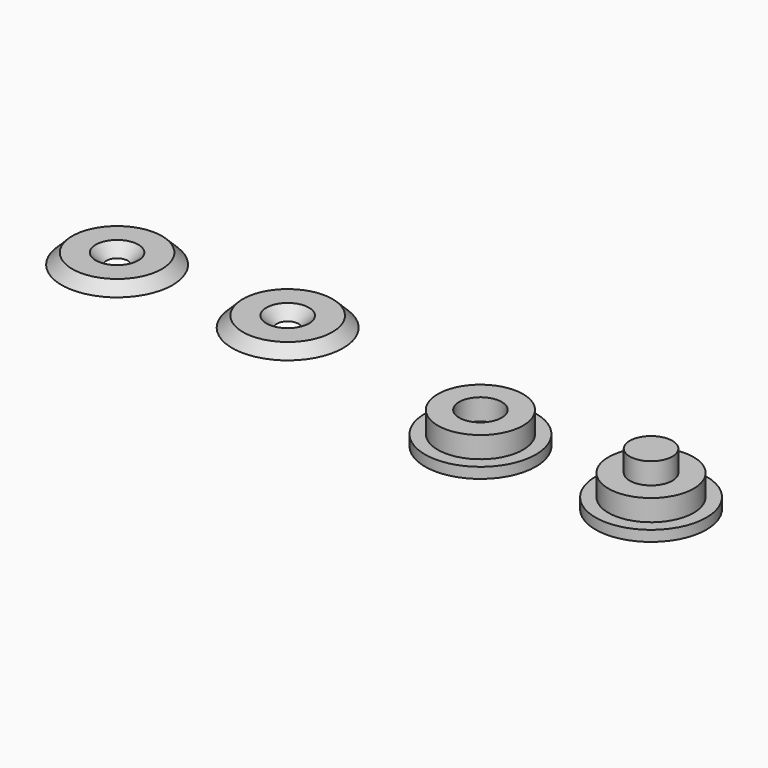
from build123d import *

# Parameters (mm, degrees)
F0_R      = 6.35
F0_R_2    = 3.175
F1_DEPTH  = 3.175
F2_R      = 8.255
F3_DEPTH  = 3.175
F5_R      = 3.175
F6_DEPTH  = 6.35
F8_DEPTH  = 3.175
F10_DEPTH = 6.35
F11_DEPTH = 1.5875
F12_R     = 8.255
F13_DEPTH = 1.5875
F13_TAPER = 45
F14_R     = 3.175
F16_DEPTH = 1.5875


# Not quite as in the source:
# - an extrude whose draft closes it to a point is written as a loft to that point


with BuildPart() as f1:
    # F0 (on Top) → F1 (new body)
    with BuildSketch(Plane.XY):
        Circle(F0_R)
        Circle(F0_R_2, mode=Mode.SUBTRACT)
    extrude(amount=F1_DEPTH)

    # F2 (on face) → F3 (join)
    with BuildSketch(Plane(origin=(0, 0, 0), x_dir=(1, 0, 0), z_dir=(0, 0, -1))):
        Circle(F2_R)
    extrude(amount=F3_DEPTH)


with BuildPart() as f4_1:
    # F4: copy of F1
    add(f1.part.moved(Location((25.4, 0, 0))))

    # F10 (add): a face of the model
    f10_faces = [f4_1.faces().sort_by_distance(p)[0] for p in [
        (25.4, 0, 0),
    ]]
    extrude(f10_faces, amount=F10_DEPTH)

    # F11 (cut): a face of the model
    f11_faces = [f4_1.faces().sort_by_distance(p)[0] for p in [
        (25.4, 0, -3.175),
    ]]
    extrude(f11_faces, amount=-F11_DEPTH, mode=Mode.SUBTRACT)


with BuildPart() as f6:
    # F5 (on Top) → F6 (new body)
    with BuildSketch(Plane.XY):
        with Locations((54.820228368, 6.1548263766)):
            Circle(F5_R)
    extrude(amount=F6_DEPTH)

    # F7 (on face) → F8 (join)
    with BuildSketch(Plane.XY.offset(6.35)):
        Polygon((54.820228368, 6.1548263766), (54.820228368, 4.8848263766), (58.630228368, 4.8848263766), (58.630228368, 7.4248263766), (54.820228368, 7.4248263766), align=None)
    extrude(amount=-F8_DEPTH)


with BuildPart() as f13:
    # F12 (on Top) → F13 (new body)
    with BuildSketch(Plane.XY):
        with Locations((-34.2364721, 6.9202007726)):
            Circle(F12_R)
    extrude(amount=F13_DEPTH, taper=F13_TAPER)

    # F14 (on face) → F15 section 0
    with BuildSketch(Plane.XY.offset(1.5875), mode=Mode.PRIVATE) as f15_s0:
        with Locations((-34.2364721, 6.9202007726)):
            Circle(F14_R)
    loft([f15_s0.sketch, Vertex(-34.2364721, 6.9202007726, -1.5875)], ruled=True, mode=Mode.SUBTRACT)


with BuildPart() as f1_1:
    add(f1.part)

    # F16 (cut): a face of the model
    f16_faces = [f1_1.faces().sort_by_distance(p)[0] for p in [
        (0, 0, -3.175),
    ]]
    extrude(f16_faces, amount=-F16_DEPTH, mode=Mode.SUBTRACT)


with BuildPart() as f17_1:
    # F17: copy of F13
    add(f13.part.moved(Location((-25.4, 0, 0))))


solid = Compound([f4_1.part, f13.part, f1_1.part, f17_1.part])
